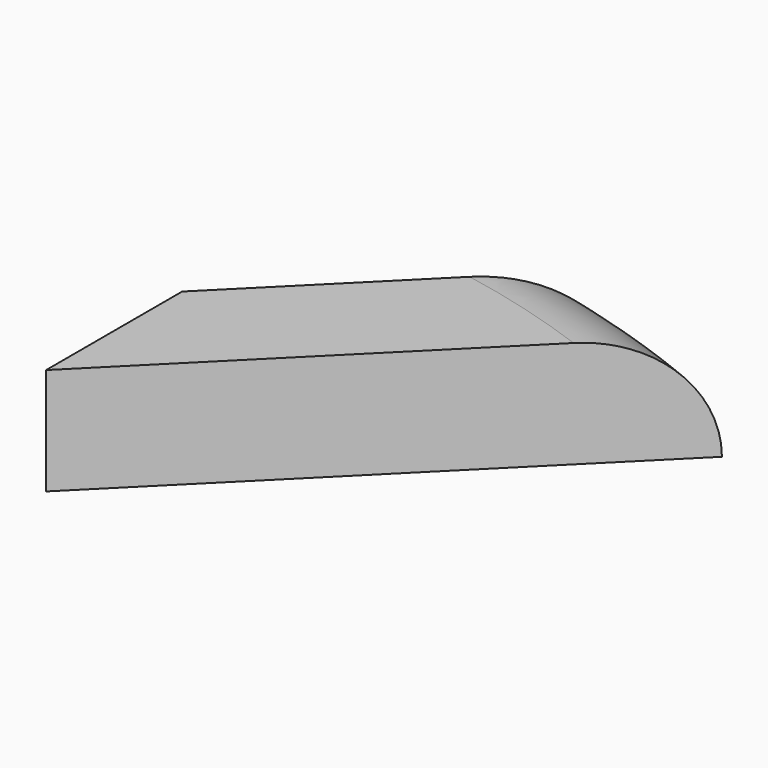
from build123d import *

# Parameters (mm, degrees)
F2_DEPTH = 25.4
F3_R     = 25.39999


# Not quite as in the source:
# - a fillet or chamfer is up to 0.001 mm smaller than in the source, because OpenCascade refuses the exact size


with BuildPart() as f2:
    # F1 (on face) → F2 (new body)
    with BuildSketch(Plane.XY):
        with BuildLine():
            Line((0, 161.6446101792), (0, 121.2334576344))
            Line((0, 121.2334576344), (89.2318353651, 210.4652929995))
            ThreePointArc((89.2318353651, 210.4652929995), (74.3790189354, 216.1613322086), (59.1660337104, 220.8106438897))
            Line((59.1660337104, 220.8106438897), (0, 161.6446101792))
        make_face()
    extrude(amount=F2_DEPTH)

    # F3 (radius 25.4 in the source; OpenCascade refuses exactly that, so slightly less here)
    f3_edges = [f2.edges().sort_by_distance(p)[0] for p in [
        (74.379019, 216.161332, 25.4),
    ]]
    fillet(f3_edges, radius=F3_R)


solid = f2.part
